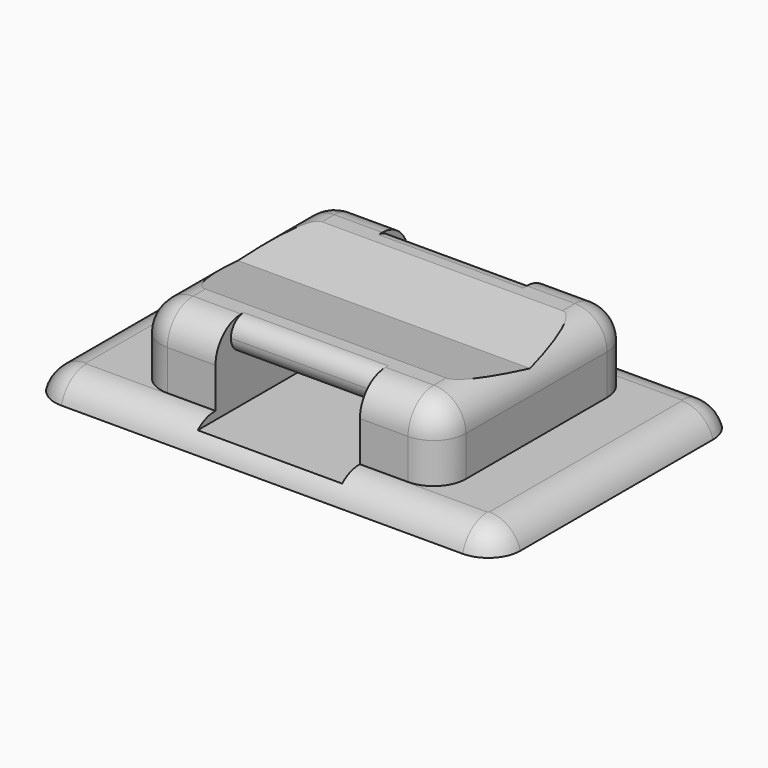
from build123d import *

# Parameters (mm, degrees)
F1_DEPTH      = 1.5
F2_W          = 19
F2_H          = 15
F3_DEPTH      = 4.5
F4_W          = 9
F4_H          = 3
F5_DEPTH      = 12.5
F6_W          = 9
F6_H          = 2
F7_DEPTH      = 1.2
F8_W          = 9
F8_H          = 2
F9_DEPTH      = 1.3
F10_R         = 2
F11_T1_DEPTH  = 8
F11_T3_DEPTH  = 2.5
F11_T5_DEPTH  = 8
F11_T7_DEPTH  = 15
F11_T9_DEPTH  = 12.8412291828
F11_T11_DEPTH = 12.8412291828
F11_T14_ANGLE = 90
F11_T16_ANGLE = 90
F11_T18_ANGLE = 90
F11_T20_ANGLE = 90
F11_T22_ANGLE = 90
F11_T24_ANGLE = 90
F11_T26_ANGLE = 90
F11_T28_ANGLE = 90
F12_T1_DEPTH  = 9
F14_DEPTH     = 12.5


# Not quite as in the source:
# - a fillet or chamfer that OpenCascade refuses, or shapes differently, is made with other operations: its cross-section is extruded or revolved along the edge and cut away or added


with BuildPart() as f1:
    # F0 (on Top) → F1 (new body)
    with BuildSketch(Plane.XY):
        with BuildLine():
            Line((12.5, 9.5), (-12.5, 9.5))
            ThreePointArc((-12.5, 9.5), (-13.9142135624, 8.9142135624), (-14.5, 7.5))
            Line((-14.5, 7.5), (-14.5, -7.5))
            ThreePointArc((-14.5, -7.5), (-13.9142135624, -8.9142135624), (-12.5, -9.5))
            Line((-12.5, -9.5), (12.5, -9.5))
            ThreePointArc((12.5, -9.5), (13.9142135624, -8.9142135624), (14.5, -7.5))
            Line((14.5, -7.5), (14.5, 7.5))
            ThreePointArc((14.5, 7.5), (13.9142135624, 8.9142135624), (12.5, 9.5))
        make_face()
    extrude(amount=F1_DEPTH)

    # F2 (on face) → F3 (join)
    with BuildSketch(Plane.XY.offset(1.5)):
        Rectangle(F2_W, F2_H)
    extrude(amount=F3_DEPTH)

    # F4 (on Front) → F5 (cut, symmetric)
    with BuildSketch(Plane.XZ):
        with Locations((0, 2.5)):
            Rectangle(F4_W, F4_H)
    extrude(amount=F5_DEPTH, both=True, mode=Mode.SUBTRACT)

    # F6 (on face) → F7 (cut)
    with BuildSketch(Plane.XZ.offset(7.5)):
        with Locations((0, 5)):
            Rectangle(F6_W, F6_H)
    extrude(amount=-F7_DEPTH, mode=Mode.SUBTRACT)

    # F8 (on face) → F9 (cut)
    with BuildSketch(Plane(origin=(0, 7.5, 0), x_dir=(-1, 0, 0), z_dir=(0, 1, 0))):
        with Locations((0, 5)):
            Rectangle(F8_W, F8_H)
    extrude(amount=-F9_DEPTH, mode=Mode.SUBTRACT)

    # F10
    f10_edges = [f1.edges().sort_by_distance(p)[0] for p in [
        (9.5, 0, 6),
        (-9.5, 0, 6),
    ]]
    fillet(f10_edges, radius=F10_R)

    # F11: fillet of radius 2 on 18 edges, made by hand

    # F11_s2 → F11_t1 (cut)
    with BuildSketch(Plane.YZ.offset(-0.5)):
        with BuildLine():
            ThreePointArc((7.5, 4), (6.9142135624, 5.4142135624), (5.5, 6))
            Line((5.5, 6), (7.5, 6))
            Line((7.5, 6), (7.5, 4))
        make_face()
        with BuildLine():
            ThreePointArc((-5.5, 6), (-6.9142135624, 5.4142135624), (-7.5, 4))
            Line((-7.5, 4), (-7.5, 6))
            Line((-7.5, 6), (-5.5, 6))
        make_face()
    extrude(amount=F11_T1_DEPTH, mode=Mode.SUBTRACT)

    # F11_s4 → F11_t3 (cut)
    with BuildSketch(Plane.XY.offset(1.5)):
        with BuildLine():
            ThreePointArc((7.5, 7.5), (8.9142135624, 6.9142135624), (9.5, 5.5))
            Line((9.5, 5.5), (9.5, 7.5))
            Line((9.5, 7.5), (7.5, 7.5))
        make_face()
        with BuildLine():
            ThreePointArc((-7.5, 7.5), (-8.9142135624, 6.9142135624), (-9.5, 5.5))
            Line((-9.5, 5.5), (-9.5, 7.5))
            Line((-9.5, 7.5), (-7.5, 7.5))
        make_face()
        with BuildLine():
            ThreePointArc((9.5, -5.5), (8.9142135624, -6.9142135624), (7.5, -7.5))
            Line((7.5, -7.5), (9.5, -7.5))
            Line((9.5, -7.5), (9.5, -5.5))
        make_face()
        with BuildLine():
            ThreePointArc((-7.5, -7.5), (-8.9142135624, -6.9142135624), (-9.5, -5.5))
            Line((-9.5, -5.5), (-9.5, -7.5))
            Line((-9.5, -7.5), (-7.5, -7.5))
        make_face()
    extrude(amount=F11_T3_DEPTH, mode=Mode.SUBTRACT)

    # F11_s6 → F11_t5 (cut)
    with BuildSketch(Plane.YZ.offset(-7.5)):
        with BuildLine():
            ThreePointArc((5.5, 6), (6.9142135624, 5.4142135624), (7.5, 4))
            Line((7.5, 4), (7.5, 6))
            Line((7.5, 6), (5.5, 6))
        make_face()
        with BuildLine():
            ThreePointArc((-5.5, 6), (-6.9142135624, 5.4142135624), (-7.5, 4))
            Line((-7.5, 4), (-7.5, 6))
            Line((-7.5, 6), (-5.5, 6))
        make_face()
    extrude(amount=F11_T5_DEPTH, mode=Mode.SUBTRACT)

    # F11_s8 → F11_t7 (cut)
    with BuildSketch(Plane.XZ.offset(-7.5)):
        with BuildLine():
            ThreePointArc((12.5635083269, 1.5), (13.7882531983, 1.0811388301), (14.5, 0))
            Line((14.5, 0), (14.5, 1.5))
            Line((14.5, 1.5), (12.5635083269, 1.5))
        make_face()
        with BuildLine():
            ThreePointArc((-12.5635083269, 1.5), (-13.7882531983, 1.0811388301), (-14.5, 0))
            Line((-14.5, 0), (-14.5, 1.5))
            Line((-14.5, 1.5), (-12.5635083269, 1.5))
        make_face()
    extrude(amount=F11_T7_DEPTH, mode=Mode.SUBTRACT)

    # F11_s10 → F11_t9 (cut)
    with BuildSketch(Plane.YZ.offset(-0.3412291828)):
        with BuildLine():
            ThreePointArc((-7.5635083269, 1.5), (-8.7882531983, 1.0811388301), (-9.5, 0))
            Line((-9.5, 0), (-9.5, 1.5))
            Line((-9.5, 1.5), (-7.5635083269, 1.5))
        make_face()
        with BuildLine():
            ThreePointArc((7.5635083269, 1.5), (8.7882531983, 1.0811388301), (9.5, 0))
            Line((9.5, 0), (9.5, 1.5))
            Line((9.5, 1.5), (7.5635083269, 1.5))
        make_face()
    extrude(amount=F11_T9_DEPTH, mode=Mode.SUBTRACT)

    # F11_s12 → F11_t11 (cut)
    with BuildSketch(Plane.YZ.offset(-12.5)):
        with BuildLine():
            ThreePointArc((-9.5, 0), (-8.7882531983, 1.0811388301), (-7.5635083269, 1.5))
            Line((-7.5635083269, 1.5), (-9.5, 1.5))
            Line((-9.5, 1.5), (-9.5, 0))
        make_face()
        with BuildLine():
            ThreePointArc((9.5, 0), (8.7882531983, 1.0811388301), (7.5635083269, 1.5))
            Line((7.5635083269, 1.5), (9.5, 1.5))
            Line((9.5, 1.5), (9.5, 0))
        make_face()
    extrude(amount=F11_T11_DEPTH, mode=Mode.SUBTRACT)

    # F11_s13 → F11_t14 (revolve, cut)
    with BuildSketch(Plane.YZ.offset(7.5)):
        with BuildLine():
            ThreePointArc((7.5, 4), (6.9142135624, 5.4142135624), (5.5, 6))
            Line((5.5, 6), (7.5, 6))
            Line((7.5, 6), (7.5, 4))
        make_face()
    revolve(axis=Axis((7.5, 7.5, 4), (0, 1, 0)), revolution_arc=F11_T14_ANGLE, mode=Mode.SUBTRACT)

    # F11_s15 → F11_t16 (revolve, cut)
    with BuildSketch(Plane.YZ.offset(-7.5)):
        with BuildLine():
            ThreePointArc((5.5, 6), (6.9142135624, 5.4142135624), (7.5, 4))
            Line((7.5, 4), (7.5, 6))
            Line((7.5, 6), (5.5, 6))
        make_face()
    revolve(axis=Axis((-7.5, 7.5, 4), (0, -1, 0)), revolution_arc=F11_T16_ANGLE, mode=Mode.SUBTRACT)

    # F11_s17 → F11_t18 (revolve, cut)
    with BuildSketch(Plane.YZ.offset(7.5)):
        with BuildLine():
            ThreePointArc((-5.5, 6), (-6.9142135624, 5.4142135624), (-7.5, 4))
            Line((-7.5, 4), (-7.5, 6))
            Line((-7.5, 6), (-5.5, 6))
        make_face()
    revolve(axis=Axis((7.5, -7.5, 4), (0, 1, 0)), revolution_arc=F11_T18_ANGLE, mode=Mode.SUBTRACT)

    # F11_s19 → F11_t20 (revolve, cut)
    with BuildSketch(Plane.YZ.offset(-7.5)):
        with BuildLine():
            ThreePointArc((-7.5, 4), (-6.9142135624, 5.4142135624), (-5.5, 6))
            Line((-5.5, 6), (-7.5, 6))
            Line((-7.5, 6), (-7.5, 4))
        make_face()
    revolve(axis=Axis((-7.5, -7.5, 4), (0, -1, 0)), revolution_arc=F11_T20_ANGLE, mode=Mode.SUBTRACT)

    # F11_s21 → F11_t22 (revolve, cut)
    with BuildSketch(Plane.YZ.offset(-12.5)):
        with BuildLine():
            ThreePointArc((7.5635083269, 1.5), (8.7882531983, 1.0811388301), (9.5, 0))
            Line((9.5, 0), (9.5, 1.5))
            Line((9.5, 1.5), (7.5635083269, 1.5))
        make_face()
    revolve(axis=Axis((-12.5, 7.5, 1.5), (0, 0, 1)), revolution_arc=F11_T22_ANGLE, mode=Mode.SUBTRACT)

    # F11_s23 → F11_t24 (revolve, cut)
    with BuildSketch(Plane.XZ.offset(-7.5)):
        with BuildLine():
            ThreePointArc((12.5635083269, 1.5), (13.7882531983, 1.0811388301), (14.5, 0))
            Line((14.5, 0), (14.5, 1.5))
            Line((14.5, 1.5), (12.5635083269, 1.5))
        make_face()
    revolve(axis=Axis((12.5, 7.5, 1.5), (0, 0, 1)), revolution_arc=F11_T24_ANGLE, mode=Mode.SUBTRACT)

    # F11_s25 → F11_t26 (revolve, cut)
    with BuildSketch(Plane.XZ.offset(7.5)):
        with BuildLine():
            ThreePointArc((-12.5635083269, 1.5), (-13.7882531983, 1.0811388301), (-14.5, 0))
            Line((-14.5, 0), (-14.5, 1.5))
            Line((-14.5, 1.5), (-12.5635083269, 1.5))
        make_face()
    revolve(axis=Axis((-12.5, -7.5, 1.5), (0, 0, 1)), revolution_arc=F11_T26_ANGLE, mode=Mode.SUBTRACT)

    # F11_s27 → F11_t28 (revolve, cut)
    with BuildSketch(Plane.YZ.offset(12.5)):
        with BuildLine():
            ThreePointArc((-7.5635083269, 1.5), (-8.7882531983, 1.0811388301), (-9.5, 0))
            Line((-9.5, 0), (-9.5, 1.5))
            Line((-9.5, 1.5), (-7.5635083269, 1.5))
        make_face()
    revolve(axis=Axis((12.5, -7.5, 1.5), (0, 0, 1)), revolution_arc=F11_T28_ANGLE, mode=Mode.SUBTRACT)

    # F12: fillet of radius 1 on 4 edges, made by hand

    # F12_s2 → F12_t1 (cut)
    with BuildSketch(Plane.YZ.offset(-4.5)):
        with BuildLine():
            ThreePointArc((-6.3, 5), (-6.0071067812, 4.2928932188), (-5.3, 4))
            Line((-5.3, 4), (-6.3, 4))
            Line((-6.3, 4), (-6.3, 5))
        make_face()
        with BuildLine():
            ThreePointArc((5.2, 4), (5.9071067812, 4.2928932188), (6.2, 5))
            Line((6.2, 5), (6.2, 4))
            Line((6.2, 4), (5.2, 4))
        make_face()
        with BuildLine():
            ThreePointArc((6.2, 5), (5.9071067812, 5.7071067812), (5.2, 6))
            Line((5.2, 6), (5.2, 6.1))
            ThreePointArc((5.2, 6.1), (5.5, 6.1), (6.235, 5.9671743695))
            Line((6.235, 5.9671743695), (6.3, 5.8734993995))
            Line((6.3, 5.8734993995), (6.3, 5))
            Line((6.3, 5), (6.2, 5))
        make_face()
        with BuildLine():
            ThreePointArc((-5.3, 6), (-6.0071067812, 5.7071067812), (-6.3, 5))
            Line((-6.3, 5), (-6.4, 5))
            Line((-6.4, 5), (-6.4, 5.833030278))
            Line((-6.4, 5.833030278), (-6.34, 5.9246817919))
            ThreePointArc((-6.34, 5.9246817919), (-5.5, 6.1), (-5.3, 6.1))
            Line((-5.3, 6.1), (-5.3, 6))
        make_face()
    extrude(amount=F12_T1_DEPTH, mode=Mode.SUBTRACT)

    # F13 (on Right) → F14 (cut, symmetric)
    with BuildSketch(Plane.YZ):
        Polygon((-10, 6.9632698071), (0, 5.2), (10, 6.9632698071), align=None)
    extrude(amount=F14_DEPTH, both=True, mode=Mode.SUBTRACT)


solid = f1.part
